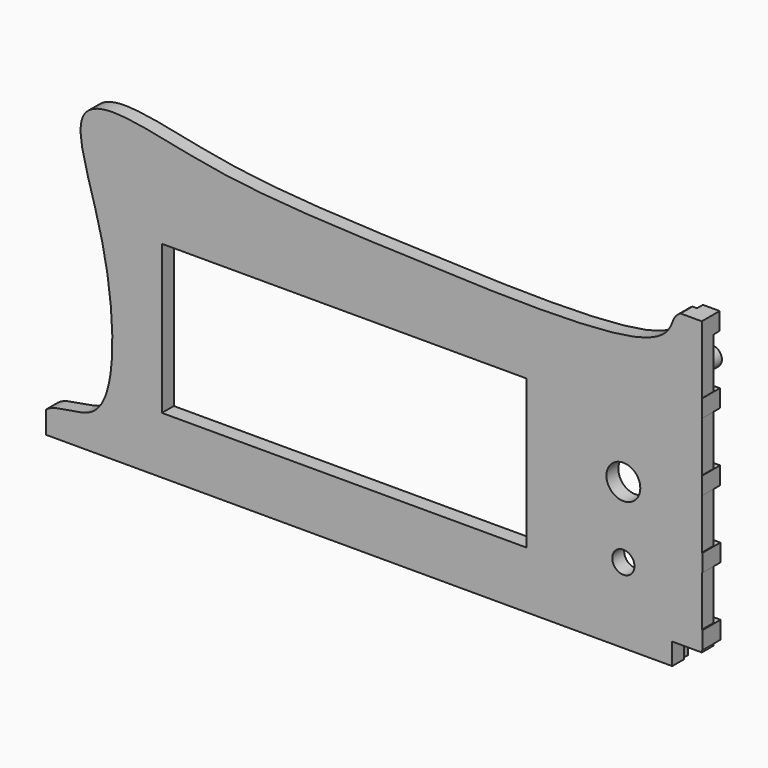
from build123d import *

# Parameters (mm, degrees)
F0_R     = 2.9777305249
F0_R_2   = 4.5459324983
F1_DEPTH = 4
F2_W     = 4.3037682772
F2_H     = 4.5
F2_W_2   = 4.5
F2_H_2   = 4.7181323171
F3_DEPTH = 6
F4_R     = 2.5211771025
F5_DEPTH = 12
F6_R     = 1.4009025459
F6_R_2   = 1.3998178409
F7_DEPTH = 9
F8_R     = 2


with BuildPart() as f1:
    # F0 (on Front) → F1 (new body)
    with BuildSketch(Plane.XZ):
        with BuildLine():
            Line((-95.4278409481, -40.3547473252), (-95.4278409481, -46.3577248156))
            Line((-95.4278409481, -46.3577248156), (-90.6878511674, -46.3577248156))
            add(Edge.make_bspline(
                [(-47.2556848285, -31.0434222525), (-66.2071872784, -39.2541441109), (-82.2106525971, -45.1740109986), (-90.6878511674, -46.3577248156)],
                knots=[0.895739685, 0.895739685, 0.895739685, 0.895739685, 0.9495042682, 0.9495042682, 0.9495042682, 0.9495042682], degree=3))
            Line((-47.2556848285, -31.0434222525), (-64.3119981289, -31.0434222525))
            Line((-64.3119981289, -31.0434222525), (-64.3119981289, 8.9565777475))
            Line((-64.3119981289, 8.9565777475), (33.6880018711, 8.9565777475))
            Line((33.6880018711, 8.9565777475), (33.6880018711, 8.3636850741))
            add(Edge.make_bspline(
                [(80.7607844472, 37.7971865237), (79.9293326803, 34.4997677685), (59.9654214438, 22.406338735), (33.6880018711, 8.3636850741)],
                knots=[0.7480183731, 0.7480183731, 0.7480183731, 0.7480183731, 0.8237972081, 0.8237972081, 0.8237972081, 0.8237972081], degree=3))
            Line((80.7607844472, 37.7971865237), (75.0439986587, 37.7971865237))
            add(Edge.make_bspline(
                [(-95.4278409481, -40.3547473252), (-92.0674179131, -37.808383953), (-76.3258009125, -41.7720249364), (-77.3177273216, -1.014959725), (-85.4659986726, 20.5289663767), (-87.0111734686, 33.1871332132), (-77.6207246502, 37.641199644), (-48.3559341751, 29.3997954409), (-2.6181687816, 27.577109738), (62.1116438555, 25.0455332175), (72.8737447638, 32.721325141), (73.1178660635, 36.728137061), (75.0439986587, 37.7971865237)],
                knots=[0, 0, 0, 0, 0.0569827595, 0.1456884161, 0.223927708, 0.2728704579, 0.3147125654, 0.3955028348, 0.5056084396, 0.6278531079, 0.6766652208, 0.7113340821, 0.7113340821, 0.7113340821, 0.7113340821], degree=3))
        make_face()
        with BuildLine():
            add(Edge.make_bspline(
                [(-47.2556848285, -31.0434222525), (-66.2071872784, -39.2541441109), (-82.2106525971, -45.1740109986), (-90.6878511674, -46.3577248156)],
                knots=[0.895739685, 0.895739685, 0.895739685, 0.895739685, 0.9495042682, 0.9495042682, 0.9495042682, 0.9495042682], degree=3))
            Line((-90.6878511674, -46.3577248156), (72.8146284819, -46.3577248156))
            Line((72.8146284819, -46.3577248156), (72.8146284819, -40.5435077846))
            Line((72.8146284819, -40.5435077846), (80.7607844472, -40.5435077846))
            Line((80.7607844472, -40.5435077846), (80.7607844472, 37.7971865237))
            add(Edge.make_bspline(
                [(80.7607844472, 37.7971865237), (79.9293326803, 34.4997677685), (59.9654214438, 22.406338735), (33.6880018711, 8.3636850741)],
                knots=[0.7480183731, 0.7480183731, 0.7480183731, 0.7480183731, 0.8237972081, 0.8237972081, 0.8237972081, 0.8237972081], degree=3))
            Line((33.6880018711, 8.3636850741), (33.6880018711, -31.0434222525))
            Line((33.6880018711, -31.0434222525), (-47.2556848285, -31.0434222525))
        make_face()
        with Locations((59.6880018711, -26.0434222525)):
            Circle(F0_R, mode=Mode.SUBTRACT)
        with Locations((59.6880018711, -7.0434222525)):
            Circle(F0_R_2, mode=Mode.SUBTRACT)
    extrude(amount=F1_DEPTH)

    # F2 (on face) → F3 (join)
    with BuildSketch(Plane.XZ.offset(4)):
        with Locations((-93.2759568095, -44.1077248156)):
            Rectangle(F2_W, F2_H)
        with Locations((-69.9340668095, -44.1077248156)):
            Rectangle(F2_W, F2_H)
        with Locations((-46.5921768095, -44.1077248156)):
            Rectangle(F2_W, F2_H)
        with Locations((-23.2502868095, -44.1077248156)):
            Rectangle(F2_W, F2_H)
        with Locations((0.0916031905, -44.1077248156)):
            Rectangle(F2_W, F2_H)
        with Locations((23.4334931905, -44.1077248156)):
            Rectangle(F2_W, F2_H)
        with Locations((46.7753831905, -44.1077248156)):
            Rectangle(F2_W, F2_H)
        with Locations((70.1172731905, -44.1077248156)):
            Rectangle(F2_W, F2_H)
        with Locations((78.5107844472, 35.4381203651)):
            Rectangle(F2_W_2, F2_H_2)
        with Locations((78.5710280145, 17.1985961585)):
            Rectangle(F2_W_2, F2_H_2)
        with Locations((78.6312715817, -1.0409280481)):
            Rectangle(F2_W_2, F2_H_2)
        with Locations((78.691515149, -19.2804522547)):
            Rectangle(F2_W_2, F2_H_2)
        with Locations((78.7517587162, -37.5199764613)):
            Rectangle(F2_W_2, F2_H_2)
    extrude(amount=-F3_DEPTH)

    # F4 (on face) → F5 (join)
    with BuildSketch(Plane(origin=(0, 0, 0), x_dir=(-1, 0, 0), z_dir=(0, 1, 0))):
        with Locations((-70.8523467183, 19.847869873)):
            Circle(F4_R)
        with Locations((74.7639298199, 19.847869873)):
            Circle(F4_R)
    extrude(amount=F5_DEPTH)

    # F6 (on face) → F7 (cut)
    with BuildSketch(Plane(origin=(0, 12, 0), x_dir=(-1, 0, 0), z_dir=(0, 1, 0))):
        with Locations((-70.8523467183, 19.847869873)):
            Circle(F6_R)
        with Locations((74.7202411294, 19.8884755373)):
            Circle(F6_R_2)
    extrude(amount=-F7_DEPTH, mode=Mode.SUBTRACT)

    # F8
    f8_edges = [f1.edges().sort_by_distance(p)[0] for p in [
        (73.373524, 0, 19.84787),
        (-72.242753, 0, 19.84787),
    ]]
    fillet(f8_edges, radius=F8_R)


solid = f1.part
